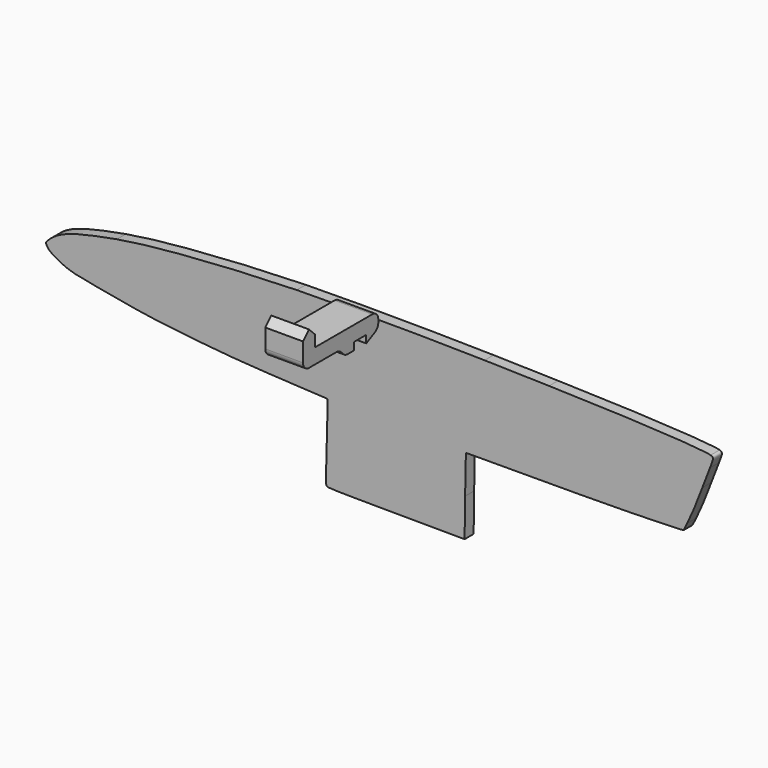
from build123d import *

# Parameters (mm, degrees)
F0_W     = 4
F0_H     = 5
F1_DEPTH = 10
F2_R     = 2
F3_SIZE  = 1.99999
F5_DEPTH = 3


# Not quite as in the source:
# - a fillet or chamfer is up to 0.001 mm smaller than in the source, because OpenCascade refuses the exact size


with BuildPart() as f1:
    # F0 (on Right) → F1 (new body)
    with BuildSketch(Plane.YZ):
        Polygon((-15.8961138576, 28.5998058021), (-15.8961138576, 32.5998058021), (-36.8961138576, 32.5998058021), (-40.8961138576, 32.5998058021), (-40.8961138576, 28.5998058021), (-28.8961138576, 28.5998058021), (-23.8961138576, 28.5998058021), (-19.8961138576, 28.5998058021), align=None)
        Polygon((-23.8961138576, 26.5998058021), (-23.8961138576, 28.5998058021), (-28.8961138576, 28.5998058021), (-26.8961138576, 26.5998058021), align=None)
        Polygon((-19.8961138576, 26.5998058021), (-15.8961138576, 28.5998058021), (-19.8961138576, 28.5998058021), align=None)
        with Locations((-38.8961138576, 35.0998058021)):
            Rectangle(F0_W, F0_H)
    extrude(amount=F1_DEPTH)

    # F2
    f2_edges = [f1.edges().sort_by_distance(p)[0] for p in [
        (5, -15.896114, 28.599806),
        (5, -26.896114, 26.599806),
        (5, -28.896114, 28.599806),
        (5, -40.896114, 28.599806),
        (5, -15.896114, 32.599806),
    ]]
    fillet(f2_edges, radius=F2_R)

    # F3 (size 2 in the source; OpenCascade refuses exactly that, so slightly less here)
    f3_edges = [f1.edges().sort_by_distance(p)[0] for p in [
        (5, -36.896114, 37.599806),
        (5, -40.896114, 37.599806),
    ]]
    chamfer(f3_edges, length=F3_SIZE)


with BuildPart() as f5:
    # F4 (on Front) → F5 (new body)
    with BuildSketch(Plane.XZ):
        with BuildLine():
            Line((-13.751079, -1.021588), (-13.881861, -6.597255))
            add(Edge.make_bspline(
                [(-14.144328, -16.709559), (-14.07191, -14.214404), (-13.9538, -9.663881), (-13.881861, -6.597255)],
                knots=[0, 0, 0, 0, 1, 1, 1, 1], degree=3))
            add(Edge.make_bspline(
                [(-13.976603, -21.494693), (-14.232522, -21.282293), (-14.256878, -20.58749), (-14.144328, -16.709559)],
                knots=[0, 0, 0, 0, 1, 1, 1, 1], degree=3))
            add(Edge.make_bspline(
                [(-6.437601, -21.79876), (-11.808741, -21.757499), (-13.754494, -21.679013), (-13.976603, -21.494693)],
                knots=[0, 0, 0, 0, 1, 1, 1, 1], degree=3))
            add(Edge.make_bspline(
                [(11.705422, -21.902138), (5.708538, -21.875891), (-2.45584, -21.829353), (-6.437601, -21.79876)],
                knots=[0, 0, 0, 0, 1, 1, 1, 1], degree=3))
            Line((11.705422, -21.902138), (22.608851, -21.949918))
            Line((22.608851, -21.949918), (22.747479, -11.831771))
            add(Edge.make_bspline(
                [(22.96733, -1.63243), (22.922682, -1.677105), (22.823735, -6.266801), (22.747479, -11.831771)],
                knots=[0, 0, 0, 0, 1, 1, 1, 1], degree=3))
            add(Edge.make_bspline(
                [(39.542721, -1.579231), (30.470942, -1.563709), (23.012006, -1.587697), (22.96733, -1.63243)],
                knots=[0, 0, 0, 0, 1, 1, 1, 1], degree=3))
            add(Edge.make_bspline(
                [(78.874564, -1.063216), (74.335359, -1.347272), (54.695232, -1.604969), (39.542721, -1.579231)],
                knots=[0, 0, 0, 0, 1, 1, 1, 1], degree=3))
            Line((78.874564, -1.063216), (80.747165, -0.946009))
            Line((80.747165, -0.946009), (81.723372, 1.000055))
            add(Edge.make_bspline(
                [(85.747268, 10.639524), (84.097425, 6.225766), (82.871029, 3.287861), (81.723372, 1.000055)],
                knots=[0, 0, 0, 0, 1, 1, 1, 1], degree=3))
            add(Edge.make_bspline(
                [(87.766907, 15.90215), (87.312416, 14.763496), (86.403576, 12.395313), (85.747268, 10.639524)],
                knots=[0, 0, 0, 0, 1, 1, 1, 1], degree=3))
            add(Edge.make_bspline(
                [(87.938103, 18.948005), (88.791769, 18.676253), (88.778278, 18.436026), (87.766907, 15.90215)],
                knots=[0, 0, 0, 0, 1, 1, 1, 1], degree=3))
            add(Edge.make_bspline(
                [(45.0504, 21.189104), (66.354481, 20.677689), (85.676176, 19.668039), (87.938103, 18.948005)],
                knots=[0, 0, 0, 0, 1, 1, 1, 1], degree=3))
            add(Edge.make_bspline(
                [(27.915476, 21.611873), (32.516714, 21.495117), (40.22742, 21.304871), (45.0504, 21.189104)],
                knots=[0, 0, 0, 0, 1, 1, 1, 1], degree=3))
            add(Edge.make_bspline(
                [(-21.977377, 21.818629), (-12.375105, 22.062694), (14.543589, 21.951132), (27.915476, 21.611873)],
                knots=[0, 0, 0, 0, 1, 1, 1, 1], degree=3))
            add(Edge.make_bspline(
                [(-69.753564, 18.150756), (-60.424959, 19.834465), (-40.817206, 21.339782), (-21.977377, 21.818629)],
                knots=[0, 0, 0, 0, 1, 1, 1, 1], degree=3))
            add(Edge.make_bspline(
                [(-87.516686, 12.458164), (-84.937485, 14.858859), (-80.998538, 16.121183), (-69.753564, 18.150756)],
                knots=[0, 0, 0, 0, 1, 1, 1, 1], degree=3))
            add(Edge.make_bspline(
                [(-88.412233, 10.73579), (-88.675914, 11.372427), (-88.669168, 11.385409), (-87.516686, 12.458164)],
                knots=[0, 0, 0, 0, 1, 1, 1, 1], degree=3))
            add(Edge.make_bspline(
                [(-85.337366, 8.232423), (-87.37628, 9.336899), (-88.065044, 9.897675), (-88.412233, 10.73579)],
                knots=[0, 0, 0, 0, 1, 1, 1, 1], degree=3))
            add(Edge.make_bspline(
                [(-74.326693, 5.15589), (-81.155143, 6.348674), (-82.610619, 6.755328), (-85.337366, 8.232423)],
                knots=[0, 0, 0, 0, 1, 1, 1, 1], degree=3))
            add(Edge.make_bspline(
                [(-64.587796, 3.439894), (-66.431131, 3.770037), (-70.813619, 4.542226), (-74.326693, 5.15589)],
                knots=[0, 0, 0, 0, 1, 1, 1, 1], degree=3))
            add(Edge.make_bspline(
                [(-51.106744, 1.728075), (-56.94022, 2.29362), (-61.22732, 2.837999), (-64.587796, 3.439894)],
                knots=[0, 0, 0, 0, 1, 1, 1, 1], degree=3))
            add(Edge.make_bspline(
                [(-46.7726, 1.23269), (-47.437855, 1.338552), (-49.388208, 1.561479), (-51.106744, 1.728075)],
                knots=[0, 0, 0, 0, 1, 1, 1, 1], degree=3))
            add(Edge.make_bspline(
                [(-28.73056, -0.174808), (-33.543126, 0.048034), (-44.890884, 0.933281), (-46.7726, 1.23269)],
                knots=[0, 0, 0, 0, 1, 1, 1, 1], degree=3))
            add(Edge.make_bspline(
                [(-14.840401, -0.91011), (-15.931302, -0.798463), (-20.608402, -0.550869), (-28.73056, -0.174808)],
                knots=[0, 0, 0, 0, 1, 1, 1, 1], degree=3))
            Line((-14.840401, -0.91011), (-13.751079, -1.021588))
        make_face()
    extrude(amount=F5_DEPTH)


solid = Compound([f1.part, f5.part])
